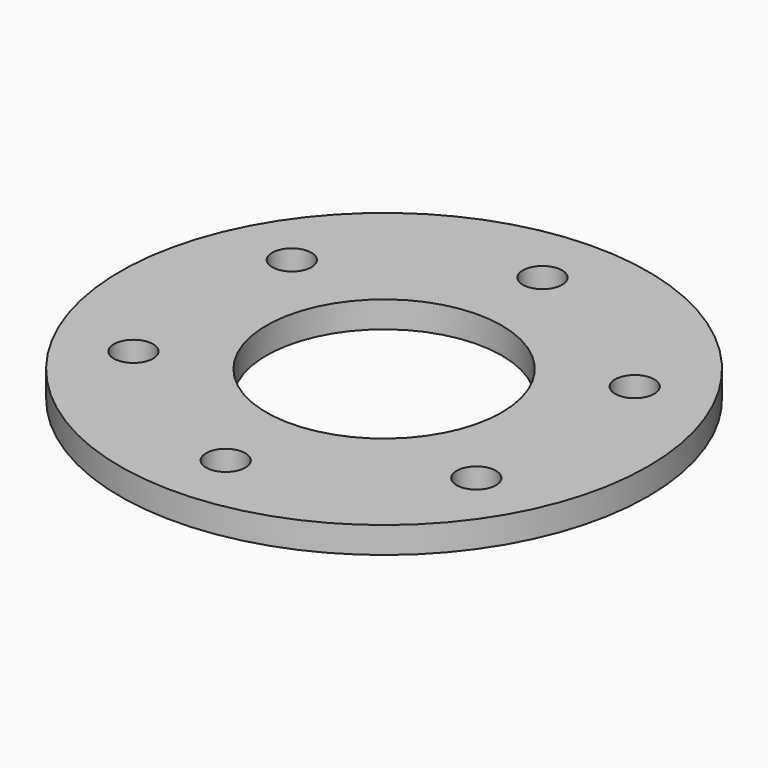
from build123d import *

# Parameters (mm, degrees)
F0_R            = 31.75
F0_R_2          = 14.1605
F1_DEPTH        = 3.175
F2_R            = 2.3622
F3_DEPTH        = 3.176
F3_COPIES_COUNT = 6


# Not quite as in the source:
# - a pattern or mirror of a feature is missing from the dataset's text; its kind, count and spacing are read off the source's solid


with BuildPart() as f1:
    # F0 (on Top) → F1 (new body)
    with BuildSketch(Plane.XY):
        Circle(F0_R)
        Circle(F0_R_2, mode=Mode.SUBTRACT)
    extrude(amount=F1_DEPTH)

    # F2 (on face) → F3 (cut, through all)
    with BuildSketch(Plane.XY.offset(3.175)):
        with Locations((0, 23.8125)):
            Circle(F2_R)
    f3 = extrude(amount=-F3_DEPTH, mode=Mode.SUBTRACT)

    # F3_copies: F3 ×6 about axis
    f3_copies_axis = Axis((0, 0, 0), (0, 0, 1))
    for i in range(1, F3_COPIES_COUNT):
        add(f3.rotate(f3_copies_axis, i * 360 / F3_COPIES_COUNT), mode=Mode.SUBTRACT)


solid = f1.part
